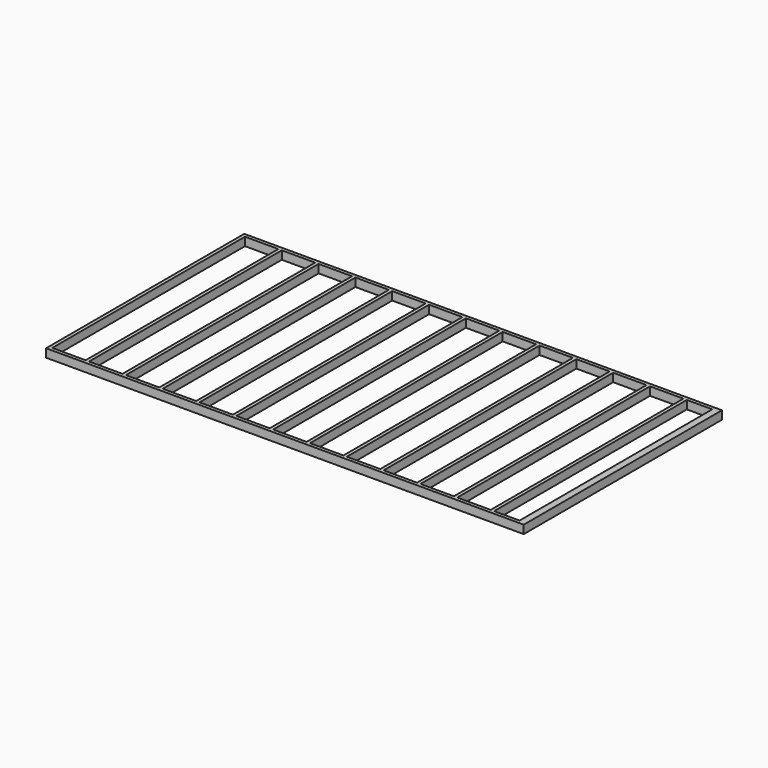
from build123d import *

# Parameters (mm, degrees)
F0_W     = 5270.6016
F0_H     = 2733.675
F0_W_2   = 38.1
F0_H_2   = 2657.475
F1_DEPTH = 92.075


# Not quite as in the source:
# - a feature names something its author has since deleted; it is built from what else it names


with BuildPart() as f1:
    # F0 (on Top) → F1 (new body)
    with BuildSketch(Plane.XY):
        with Locations((-2940.1008, 147.6375)):
            Rectangle(F0_W, F0_H)
        Polygon((-5537.3016, -1181.1), (-5537.3016, 1476.375), (-5169.1032, 1476.375), (-5131.0032, 1476.375), (-4762.8048, 1476.375), (-4724.7048, 1476.375), (-4356.5064, 1476.375), (-4318.4064, 1476.375), (-3950.208, 1476.375), (-3912.108, 1476.375), (-3543.9096, 1476.375), (-3505.8096, 1476.375), (-3137.6112, 1476.375), (-3099.5112, 1476.375), (-2731.3128, 1476.375), (-2693.2128, 1476.375), (-2325.0144, 1476.375), (-2286.9144, 1476.375), (-1918.716, 1476.375), (-1880.616, 1476.375), (-1512.4176, 1476.375), (-1474.3176, 1476.375), (-1106.1192, 1476.375), (-1068.0192, 1476.375), (-699.8208, 1476.375), (-661.7208, 1476.375), (-381, 1476.375), (-342.9, 1476.375), (-342.9, -1181.1), (-381, -1181.1), (-661.7208, -1181.1), (-699.8208, -1181.1), (-1068.0192, -1181.1), (-1106.1192, -1181.1), (-1474.3176, -1181.1), (-1512.4176, -1181.1), (-1880.616, -1181.1), (-1918.716, -1181.1), (-2286.9144, -1181.1), (-2325.0144, -1181.1), (-2693.2128, -1181.1), (-2731.3128, -1181.1), (-3099.5112, -1181.1), (-3137.6112, -1181.1), (-3505.8096, -1181.1), (-3543.9096, -1181.1), (-3912.108, -1181.1), (-3950.208, -1181.1), (-4318.4064, -1181.1), (-4356.5064, -1181.1), (-4724.7048, -1181.1), (-4762.8048, -1181.1), (-5131.0032, -1181.1), (-5169.1032, -1181.1), align=None, mode=Mode.SUBTRACT)
        with Locations((-5150.0532, 147.6375)):
            Rectangle(F0_W_2, F0_H_2)
        with Locations((-4743.7548, 147.6375)):
            Rectangle(F0_W_2, F0_H_2)
        with Locations((-4337.4564, 147.6375)):
            Rectangle(F0_W_2, F0_H_2)
        with Locations((-3931.158, 147.6375)):
            Rectangle(F0_W_2, F0_H_2)
        with Locations((-3524.8596, 147.6375)):
            Rectangle(F0_W_2, F0_H_2)
        with Locations((-3118.5612, 147.6375)):
            Rectangle(F0_W_2, F0_H_2)
        with Locations((-2712.2628, 147.6375)):
            Rectangle(F0_W_2, F0_H_2)
        with Locations((-2305.9644, 147.6375)):
            Rectangle(F0_W_2, F0_H_2)
        with Locations((-1899.666, 147.6375)):
            Rectangle(F0_W_2, F0_H_2)
        with Locations((-1493.3676, 147.6375)):
            Rectangle(F0_W_2, F0_H_2)
        with Locations((-1087.0692, 147.6375)):
            Rectangle(F0_W_2, F0_H_2)
        with Locations((-361.95, 147.6375)):
            Rectangle(F0_W_2, F0_H_2)
        with Locations((-680.7708, 147.6375)):
            Rectangle(F0_W_2, F0_H_2)
    extrude(amount=F1_DEPTH)


solid = f1.part
